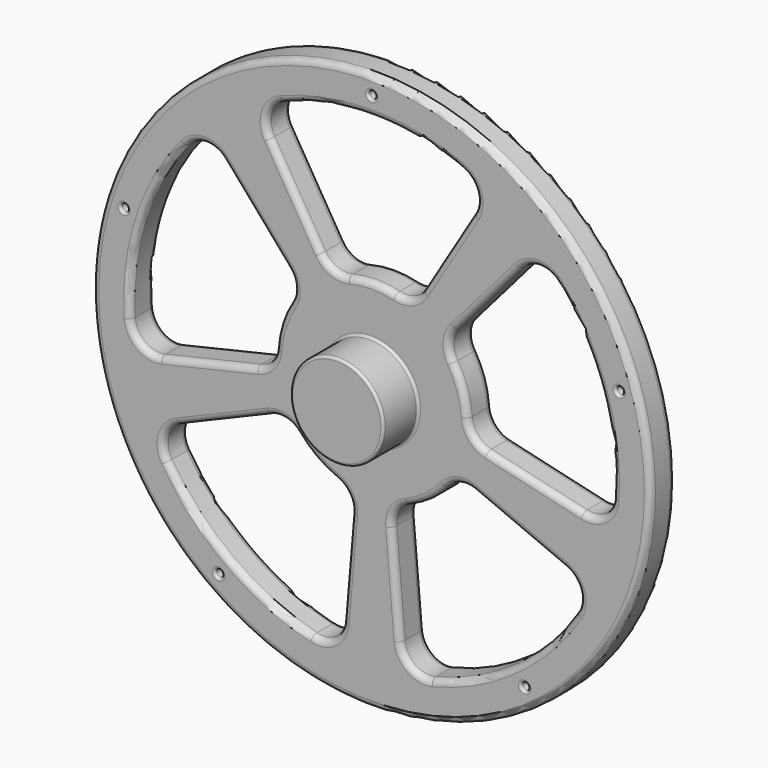
from build123d import *

# Parameters (mm, degrees)
F0_R      = 57.15
F1_DEPTH  = 6.35
F2_R      = 9.525
F3_DEPTH  = 8.89
F4_R      = 0.762
F5_DEPTH  = 15.241
F7_DEPTH  = 25.4
F8_R      = 5.08
F9_R      = 1.27
F10_R     = 0.508
F11_W     = 12.7
F11_H     = 12.7
F12_DEPTH = 3.175


with BuildPart() as f1:
    # F0 (on Front) → F1 (new body)
    with BuildSketch(Plane.XZ):
        Circle(F0_R)
    extrude(amount=F1_DEPTH)

    # F2 (on face) → F3 (join)
    with BuildSketch(Plane.XZ.offset(6.35)):
        Circle(F2_R)
    extrude(amount=F3_DEPTH)

    # F4 (on face) → F5 (cut, through all)
    with BuildSketch(Plane(origin=(0, 0, 0), x_dir=(-1, 0, 0), z_dir=(0, 1, 0))):
        with Locations((0, 53.34)):
            Circle(F4_R)
        with Locations((-50.7293545792, 16.48296648)):
            Circle(F4_R)
        with Locations((-31.3524653573, -43.15296648)):
            Circle(F4_R)
        with Locations((31.3524653573, -43.15296648)):
            Circle(F4_R)
        with Locations((50.7293545792, 16.48296648)):
            Circle(F4_R)
    extrude(amount=-F5_DEPTH, mode=Mode.SUBTRACT)

    # F6 (on face) → F7 (cut)
    with BuildSketch(Plane.XZ.offset(6.35)):
        with BuildLine():
            ThreePointArc((-19.5448914879, -2.3444491308), (-18.7215475233, 6.0829995343), (-14.4341167431, 13.3848981635))
            Line((-14.4341167431, 13.3848981635), (-34.0100114087, 36.0074995519))
            ThreePointArc((-34.0100114087, 36.0074995519), (-47.1058292521, 15.3056117314), (-48.6793544171, -9.1400959261))
            Line((-48.6793544171, -9.1400959261), (-19.5448914879, -2.3444491308))
        make_face()
        with BuildLine():
            Line((-6.35, -49.1212621988), (-3.81, -19.3127710337))
            ThreePointArc((-3.81, -19.3127710337), (-11.5705526914, -15.9254995343), (-17.1901819907, -9.591499785))
            Line((-17.1901819907, -9.591499785), (-44.7548385885, -21.218513683))
            ThreePointArc((-44.7548385885, -21.218513683), (-29.113003546, -40.0706117314), (-6.35, -49.1212621988))
        make_face()
        with BuildLine():
            ThreePointArc((17.1901819907, -9.591499785), (11.5705526914, -15.9254995343), (3.81, -19.3127710337))
            Line((3.81, -19.3127710337), (6.35, -49.1212621988))
            ThreePointArc((6.35, -49.1212621988), (29.113003546, -40.0706117314), (44.7548385885, -21.218513683))
            Line((44.7548385885, -21.218513683), (17.1901819907, -9.591499785))
        make_face()
        with BuildLine():
            ThreePointArc((14.4341167431, 13.3848981635), (18.7215475233, 6.0829995343), (19.5448914879, -2.3444491308))
            Line((19.5448914879, -2.3444491308), (48.6793544171, -9.1400959261))
            ThreePointArc((48.6793544171, -9.1400959261), (47.1058292521, 15.3056117314), (34.0100114087, 36.0074995519))
            Line((34.0100114087, 36.0074995519), (14.4341167431, 13.3848981635))
        make_face()
        with BuildLine():
            ThreePointArc((-8.2694072459, 17.863821786), (0, 19.685), (8.2694072459, 17.863821786))
            Line((8.2694072459, 17.863821786), (23.7354955801, 43.472372256))
            ThreePointArc((23.7354955801, 43.472372256), (0, 49.53), (-23.7354955801, 43.472372256))
            Line((-23.7354955801, 43.472372256), (-8.2694072459, 17.863821786))
        make_face()
    extrude(amount=-F7_DEPTH, mode=Mode.SUBTRACT)

    # F8
    f8_edges = [f1.edges().sort_by_distance(p)[0] for p in [
        (-8.269407, -3.175, 17.863822),
        (8.269407, -3.175, 17.863822),
        (-23.735496, -3.175, 43.472372),
        (23.735496, -3.175, 43.472372),
        (34.010011, -3.175, 36.0075),
        (14.434117, -3.175, 13.384898),
        (19.544891, -3.175, -2.344449),
        (48.679354, -3.175, -9.140096),
        (44.754839, -3.175, -21.218514),
        (6.35, -3.175, -49.121262),
        (3.81, -3.175, -19.312771),
        (17.190182, -3.175, -9.5915),
        (-17.190182, -3.175, -9.5915),
        (-3.81, -3.175, -19.312771),
        (-6.35, -3.175, -49.121262),
        (-44.754839, -3.175, -21.218514),
        (-48.679354, -3.175, -9.140096),
        (-19.544891, -3.175, -2.344449),
        (-14.434117, -3.175, 13.384898),
        (-34.010011, -3.175, 36.0075),
    ]]
    fillet(f8_edges, radius=F8_R)

    # F9
    f9_edges = [f1.edges().sort_by_distance(p)[0] for p in [
        (-57.15, -6.35, 0),
        (34.219281, -6.35, 33.508793),
        (7.982638, -6.35, 19.316873),
        (17.812263, -6.35, -10.935602),
        (-17.812263, -6.35, -10.935602),
        (-15.904667, -6.35, 13.561182),
        (0, 0, 49.53),
        (23.728541, 0, 24.125866),
        (30.277584, 0, -15.111881),
        (-4.896083, 0, -20.319755),
        (-23.728541, 0, 24.125866),
        (-57.15, 0, 0),
        (-29.113004, 0, -40.070612),
        (-42.443096, 0, -22.189684),
        (-7.988006, 0, -47.222772),
        (-30.277584, 0, -15.111881),
        (-5.015965, 0, -33.465522),
        (-17.812263, 0, -10.935602),
        (-11.570553, 0, -15.9255),
        (29.113004, 0, -40.070612),
        (7.988006, 0, -47.222772),
        (42.443096, 0, -22.189684),
        (5.015965, 0, -33.465522),
        (4.896083, 0, -20.319755),
        (17.812263, 0, -10.935602),
        (11.570553, 0, -15.9255),
        (-47.105829, 0, 15.305612),
        (-34.219281, 0, 33.508793),
        (-47.379955, 0, -6.995594),
        (-33.377621, 0, -5.570949),
        (-15.904667, 0, 13.561182),
        (-20.838208, 0, -1.622698),
        (-18.721548, 0, 6.083),
        (34.219281, 0, 33.508793),
        (15.904667, 0, 13.561182),
        (47.105829, 0, 15.305612),
        (18.721548, 0, 6.083),
        (47.379955, 0, -6.995594),
        (20.838208, 0, -1.622698),
        (33.377621, 0, -5.570949),
        (21.294417, 0, 42.899257),
        (-21.294417, 0, 42.899257),
        (15.612539, 0, 30.022486),
        (-15.612539, 0, 30.022486),
        (7.982638, 0, 19.316873),
        (-7.982638, 0, 19.316873),
        (0, 0, 19.685),
        (-29.113004, -6.35, -40.070612),
        (-42.443096, -6.35, -22.189684),
        (-7.988006, -6.35, -47.222772),
        (-30.277584, -6.35, -15.111881),
        (-5.015965, -6.35, -33.465522),
        (-4.896083, -6.35, -20.319755),
        (-11.570553, -6.35, -15.9255),
        (29.113004, -6.35, -40.070612),
        (7.988006, -6.35, -47.222772),
        (42.443096, -6.35, -22.189684),
        (5.015965, -6.35, -33.465522),
        (30.277584, -6.35, -15.111881),
        (4.896083, -6.35, -20.319755),
        (11.570553, -6.35, -15.9255),
        (-47.105829, -6.35, 15.305612),
        (-34.219281, -6.35, 33.508793),
        (-47.379955, -6.35, -6.995594),
        (-23.728541, -6.35, 24.125866),
        (-33.377621, -6.35, -5.570949),
        (-20.838208, -6.35, -1.622698),
        (-18.721548, -6.35, 6.083),
        (23.728541, -6.35, 24.125866),
        (15.904667, -6.35, 13.561182),
        (47.105829, -6.35, 15.305612),
        (18.721548, -6.35, 6.083),
        (47.379955, -6.35, -6.995594),
        (20.838208, -6.35, -1.622698),
        (33.377621, -6.35, -5.570949),
        (0, -6.35, 49.53),
        (21.294417, -6.35, 42.899257),
        (-21.294417, -6.35, 42.899257),
        (15.612539, -6.35, 30.022486),
        (-15.612539, -6.35, 30.022486),
        (-7.982638, -6.35, 19.316873),
        (0, -6.35, 19.685),
    ]]
    fillet(f9_edges, radius=F9_R)

    # F10
    f10_edges = [f1.edges().sort_by_distance(p)[0] for p in [
        (51.491355, 0, 16.482966),
        (0.762, 0, 53.34),
        (-49.967355, 0, 16.482966),
        (-30.590465, 0, -43.152966),
        (32.114465, 0, -43.152966),
        (-30.590465, -6.35, -43.152966),
        (32.114465, -6.35, -43.152966),
        (51.491355, -6.35, 16.482966),
        (0.762, -6.35, 53.34),
        (-49.967355, -6.35, 16.482966),
        (-9.525, -6.35, 0),
        (-9.525, -15.24, 0),
    ]]
    fillet(f10_edges, radius=F10_R)

    # F11 (on face) → F12 (cut)
    with BuildSketch(Plane(origin=(0, 0, 0), x_dir=(-1, 0, 0), z_dir=(0, 1, 0))):
        Rectangle(F11_W, F11_H)
    extrude(amount=-F12_DEPTH, mode=Mode.SUBTRACT)


solid = f1.part
